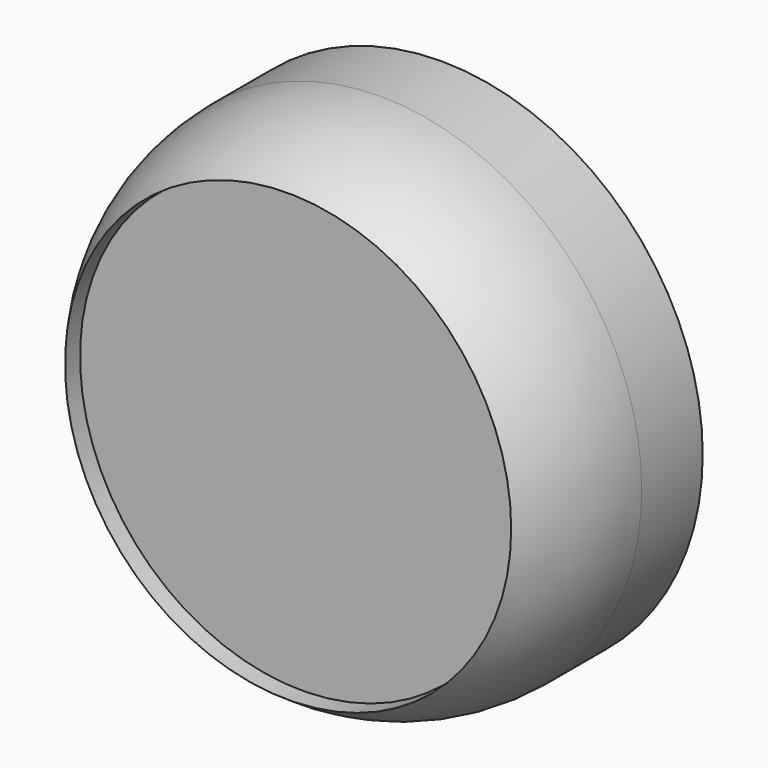
from build123d import *

# Parameters (mm, degrees)
F0_R     = 65.0568938339
F1_DEPTH = 55.88
F3_R     = 64.7387933721
F4_DEPTH = 50.8


# Not quite as in the source:
# - a fillet or chamfer that OpenCascade refuses, or shapes differently, is made with other operations: its cross-section is extruded or revolved along the edge and cut away or added


with BuildPart() as f1:
    # F0 (on Front) → F1 (new body)
    with BuildSketch(Plane.XZ):
        with BuildLine():
            ThreePointArc((76.2, 0), (53.8815367004, 53.8815367525), (-7.37e-08, 76.2))
            ThreePointArc((-7.37e-08, 76.2), (-53.8815367525, 53.8815367004), (-76.2, 0))
            ThreePointArc((-76.2, 0), (-53.8815367264, -53.8815367264), (0, -76.2))
            ThreePointArc((0, -76.2), (53.8815367264, -53.8815367264), (76.2, 0))
        make_face()
        Circle(F0_R, mode=Mode.SUBTRACT)
    extrude(amount=F1_DEPTH)

    # F2: fillet of radius 56.4153425255 on 2 edges, made by hand

    # F2_s1 → F2_t2 (revolve, cut)
    with BuildSketch(Plane.XY):
        with BuildLine():
            ThreePointArc((76.2, -22.2182191901), (73.3418212968, -39.9473216937), (65.0568938339, -55.88))
            Line((65.0568938339, -55.88), (76.2, -55.88))
            Line((76.2, -55.88), (76.2, -22.2182191901))
        make_face()
    revolve(axis=Axis((0, -55.88, 0), (0, 1, 0)), mode=Mode.SUBTRACT)

    # F2_s3 → F2_t4 (revolve, cut)
    with BuildSketch(Plane.XY):
        with BuildLine():
            ThreePointArc((65.0568938339, -33.6617808099), (67.9150725371, -15.9326783063), (76.2, 0))
            Line((76.2, 0), (65.0568938339, 0))
            Line((65.0568938339, 0), (65.0568938339, -33.6617808099))
        make_face()
    revolve(axis=Axis((0, 0, 0), (0, -1, 0)), mode=Mode.SUBTRACT)


with BuildPart() as f4:
    # F3 (on face) → F4 (new body)
    with BuildSketch(Plane.XZ):
        Circle(F3_R)
    extrude(amount=F4_DEPTH)


solid = Compound([f1.part, f4.part])
